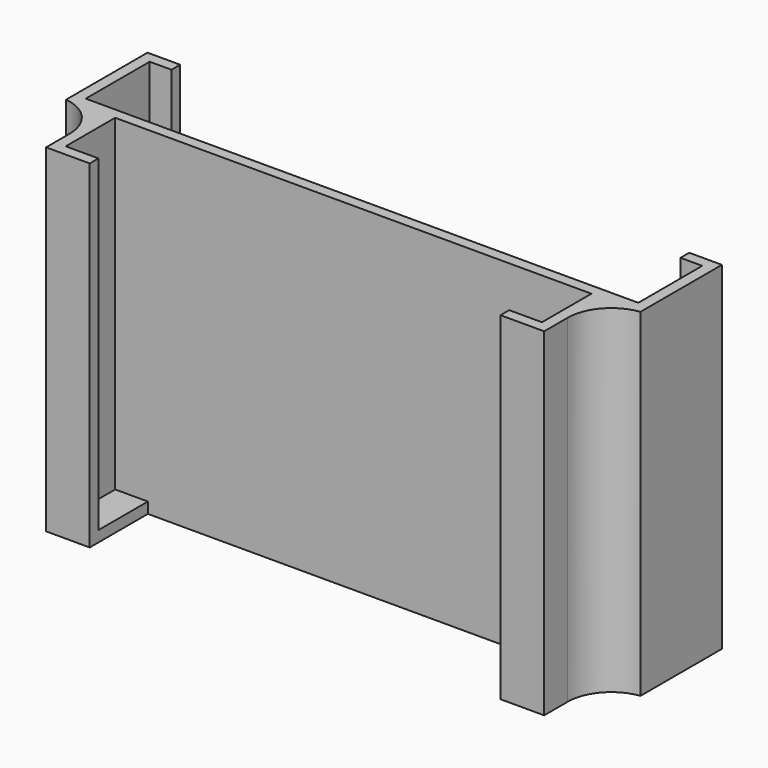
from build123d import *

# Parameters (mm, degrees)
F1_DEPTH    = 45
F2_T1_DEPTH = 45
F3_W        = 4.5
F3_H        = 8.5
F4_DEPTH    = 1.5


# Not quite as in the source:
# - a fillet or chamfer that OpenCascade refuses, or shapes differently, is made with other operations: its cross-section is extruded or revolved along the edge and cut away or added


with BuildPart() as f1:
    # F0 (on Top) → F1 (new body)
    with BuildSketch(Plane.XY):
        Polygon((38, 0), (0, 0), (-38, 0), (-38, 11), (-35, 11), (-35, 12.5), (-39.5, 12.5), (-39.5, -1.5), (-34.25, -1.5), (-32.75, -1.5), (0, -1.5), (32.75, -1.5), (34.25, -1.5), (39.5, -1.5), (39.5, 12.5), (35, 12.5), (35, 11), (38, 11), align=None)
        Polygon((-32.75, -1.5), (-34.25, -1.5), (-34.25, -11.5), (-28.25, -11.5), (-28.25, -10), (-32.75, -10), align=None)
        Polygon((34.25, -11.5), (34.25, -1.5), (32.75, -1.5), (32.75, -10), (28.25, -10), (28.25, -11.5), align=None)
    extrude(amount=F1_DEPTH)

    # F2: fillet of radius 6 on 2 edges, made by hand

    # F2_s2 → F2_t1 (join)
    with BuildSketch(Plane.XY):
        with BuildLine():
            ThreePointArc((-39.5, -1.5), (-35.75, -3.4843134833), (-34.25, -7.4529404499))
            Line((-34.25, -7.4529404499), (-34.25, -1.5))
            Line((-34.25, -1.5), (-39.5, -1.5))
        make_face()
        with BuildLine():
            ThreePointArc((34.25, -7.4529404499), (35.75, -3.4843134833), (39.5, -1.5))
            Line((39.5, -1.5), (34.25, -1.5))
            Line((34.25, -1.5), (34.25, -7.4529404499))
        make_face()
    extrude(amount=F2_T1_DEPTH)

    # F3 (on face) → F4 (join)
    with BuildSketch(Plane(origin=(0, 0, 0), x_dir=(1, 0, 0), z_dir=(0, 0, -1))):
        with BuildLine():
            Line((-39.5, -12.5), (-35, -12.5))
            Line((-35, -12.5), (-35, -11))
            Line((-35, -11), (-38, -11))
            Line((-38, -11), (-38, 0))
            Line((-38, 0), (-20, 0))
            Line((-20, 0), (20, 0))
            Line((20, 0), (38, 0))
            Line((38, 0), (38, -11))
            Line((38, -11), (35, -11))
            Line((35, -11), (35, -12.5))
            Line((35, -12.5), (39.5, -12.5))
            Line((39.5, -12.5), (39.5, 1.5))
            ThreePointArc((39.5, 1.5), (35.75, 3.4843134833), (34.25, 7.4529404499))
            Line((34.25, 7.4529404499), (34.25, 11.5))
            Line((34.25, 11.5), (28.25, 11.5))
            Line((28.25, 11.5), (28.25, 10))
            Line((28.25, 10), (32.75, 10))
            Line((32.75, 10), (32.75, 1.5))
            Line((32.75, 1.5), (28.25, 1.5))
            Line((28.25, 1.5), (-28.25, 1.5))
            Line((-28.25, 1.5), (-32.75, 1.5))
            Line((-32.75, 1.5), (-32.75, 10))
            Line((-32.75, 10), (-28.25, 10))
            Line((-28.25, 10), (-28.25, 11.5))
            Line((-28.25, 11.5), (-34.25, 11.5))
            Line((-34.25, 11.5), (-34.25, 7.4529404499))
            ThreePointArc((-34.25, 7.4529404499), (-35.75, 3.4843134833), (-39.5, 1.5))
            Line((-39.5, 1.5), (-39.5, -12.5))
        make_face()
        with Locations((-30.5, 5.75)):
            Rectangle(F3_W, F3_H)
        Polygon((-35, -11), (-35, -12.5), (-20, -12.5), (-20, 0), (-38, 0), (-38, -11), align=None)
        Polygon((38, 0), (20, 0), (20, -12.5), (35, -12.5), (35, -11), (38, -11), align=None)
        with Locations((30.5, 5.75)):
            Rectangle(F3_W, F3_H)
    extrude(amount=F4_DEPTH)


solid = f1.part
